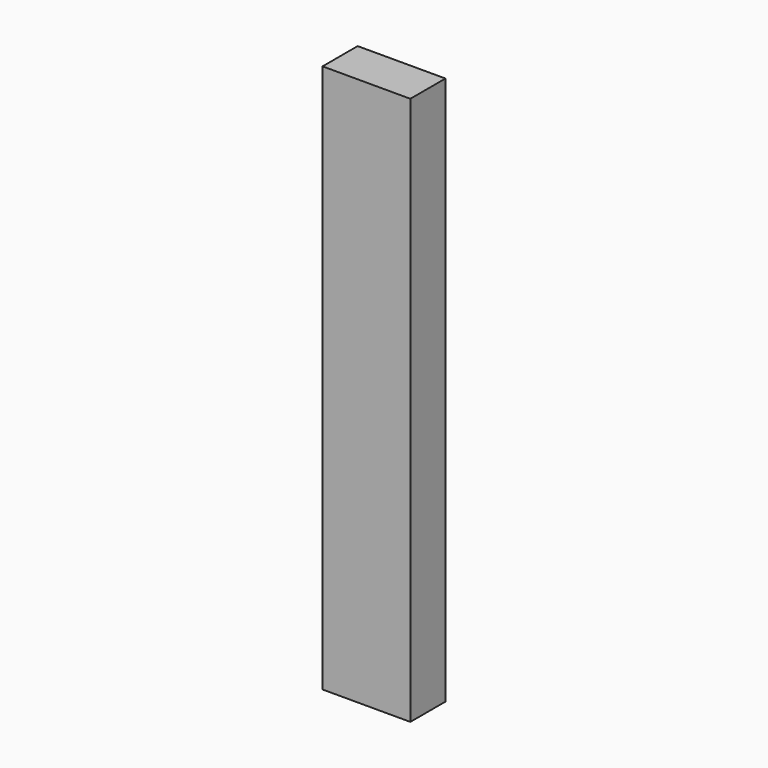
from build123d import *

# Parameters (mm, degrees)
F1_DEPTH = 10


# Not quite as in the source:
# - the program builds the solid bodies; features that only make, move or delete a surface that nothing else refers to are left out


with BuildPart() as f1:
    # F0 (on Front) → F1 (new body, symmetric)
    with BuildSketch(Plane.XZ):
        Polygon((0, -125), (0, 0), (0, 125), (-20, 125), (-20, -125), align=None)
        Polygon((0, 125), (0, 0), (0, -125), (20, -125), (20, 125), align=None)
    extrude(amount=F1_DEPTH, both=True)


solid = f1.part
